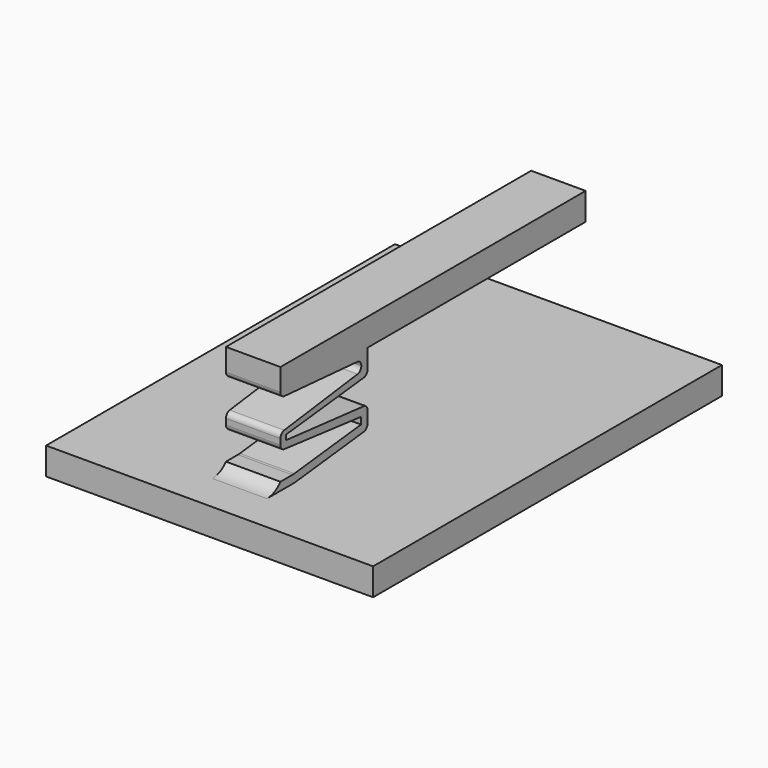
from build123d import *

# Parameters (mm, degrees)
F0_W        = 76.2
F0_H        = 101.6
F1_DEPTH    = 6.35
F2_W        = 12.7
F2_H        = 25.4
F3_DEPTH    = 25.4
F4_W        = 63.5
F4_H        = 6.35
F5_DEPTH    = 12.7
F7_DEPTH    = 12.7
F8_T1_DEPTH = 12.7
F9_R        = 1.27


# Not quite as in the source:
# - a fillet or chamfer that OpenCascade refuses, or shapes differently, is made with other operations: its cross-section is extruded or revolved along the edge and cut away or added


with BuildPart() as f1:
    # F0 (on Top) → F1 (new body)
    with BuildSketch(Plane.XY):
        Rectangle(F0_W, F0_H)
    extrude(amount=-F1_DEPTH)

    # F2 (on face) → F3 (join)
    with BuildSketch(Plane.XY):
        with Locations((0, -25.4)):
            Rectangle(F2_W, F2_H)
    extrude(amount=F3_DEPTH)

    # F4 (on face) → F5 (join, through all)
    with BuildSketch(Plane.YZ.offset(6.35)):
        with Locations((19.05, 22.225)):
            Rectangle(F4_W, F4_H)
    extrude(amount=-F5_DEPTH)

    # F6 (on face) → F7 (cut, through all)
    with BuildSketch(Plane.YZ.offset(6.35)):
        Polygon((-12.7, 2.3706669454), (-33.9936651289, 0), (-12.7, 0), align=None)
        Polygon((-38.1, 1.8626668025), (-34.33233127, 1.8626668025), (-14.6236953676, 4.0568692279), (-14.6236953676, 5.64925652), (-38.1, 8.2224374637), align=None)
        Polygon((-36.4234596491, 9.7253257409), (-12.7, 7.3805158027), (-12.7, 13.4764490649), (-36.4234596491, 10.8793787658), align=None)
        Polygon((-38.1, 19.05), (-38.1, 11.84564922), (-14.5409666002, 14.9470388849), (-14.5409666002, 17.2827038914), align=None)
    extrude(amount=-F7_DEPTH, mode=Mode.SUBTRACT)

    # F8: fillet of radius 5.08 on 2 edges, made by hand

    # F8_s2 → F8_t1 (join)
    with BuildSketch(Plane.YZ.offset(-6.35)):
        with BuildLine():
            ThreePointArc((-42.0313060293, 0), (-39.8561799, 0.4892237779), (-38.1, 1.8626668025))
            Line((-38.1, 1.8626668025), (-38.1, 0))
            Line((-38.1, 0), (-42.0313060293, 0))
        make_face()
        with BuildLine():
            ThreePointArc((-34.6142437504, 1.8626668025), (-34.3327643656, 1.870471089), (-34.0521498413, 1.8938599694))
            Line((-34.0521498413, 1.8938599694), (-34.33233127, 1.8626668025))
            Line((-34.33233127, 1.8626668025), (-34.6142437504, 1.8626668025))
        make_face()
    extrude(amount=F8_T1_DEPTH)

    # F9
    f9_edges = [f1.edges().sort_by_distance(p)[0] for p in [
        (0, -12.7, 7.380516),
        (0, -12.7, 2.370667),
        (0, -38.1, 11.845649),
        (0, -38.1, 8.222437),
        (0, -12.7, 13.476449),
        (0, -38.1, 19.05),
        (0, -14.540967, 17.282704),
        (0, -14.540967, 14.947039),
    ]]
    fillet(f9_edges, radius=F9_R)


solid = f1.part
